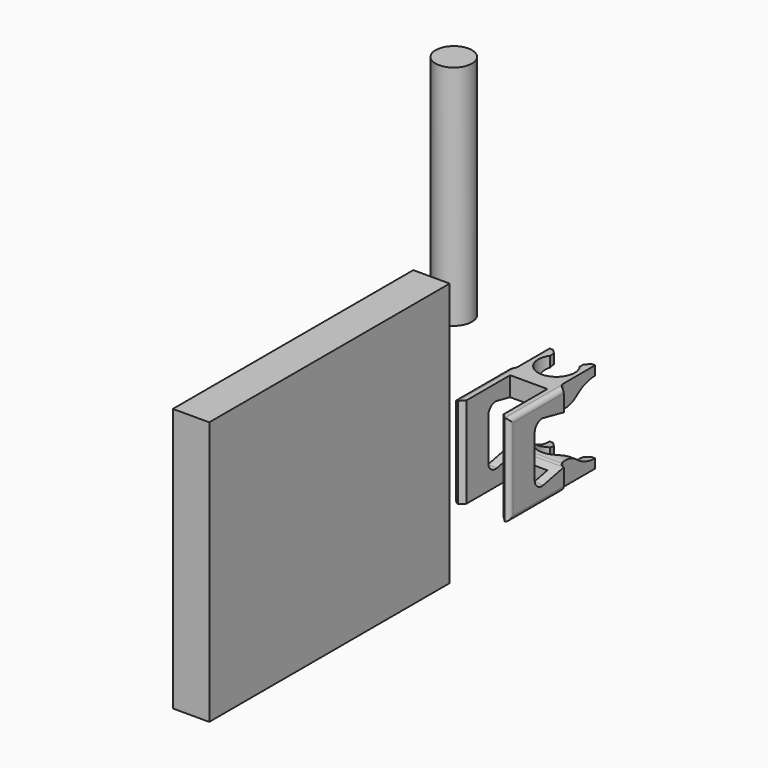
from build123d import *

# Parameters (mm, degrees)
F0_W        = 2
F0_H        = 20
F0_W_2      = 8.2
F1_DEPTH    = 15
F2_DEPTH    = 13
F3_W        = 10
F3_H        = 20
F4_DEPTH    = 10
F5_T1_DEPTH = 20
F7_DEPTH    = 20.001
F8_SIZE     = 1
F9_R        = 1
F10_SIZE    = 0.99999
F11_R       = 4
F12_DEPTH   = 50
F13_W       = 66.0741459578
F13_H       = 57.9895451665
F14_DEPTH   = 8
F16_DEPTH   = 25


# Not quite as in the source:
# - a fillet or chamfer that OpenCascade refuses, or shapes differently, is made with other operations: its cross-section is extruded or revolved along the edge and cut away or added
# - a fillet or chamfer is up to 0.001 mm smaller than in the source, because OpenCascade refuses the exact size
# - a feature names something its author has since deleted; it is built from what else it names


with BuildPart() as f1:
    # F0 (on Front) → F1 (new body)
    with BuildSketch(Plane.XZ):
        with Locations((1, 10)):
            Rectangle(F0_W, F0_H)
        with Locations((-9.2, 10)):
            Rectangle(F0_W, F0_H)
        with Locations((-4.1, 10)):
            Rectangle(F0_W_2, F0_H)
    extrude(amount=-F1_DEPTH)

    # F0 (on Front) → F2 (cut)
    with BuildSketch(Plane.XZ):
        with Locations((-4.1, 10)):
            Rectangle(F0_W_2, F0_H)
    extrude(amount=-F2_DEPTH, mode=Mode.SUBTRACT)

    # F3 (on face) → F4 (join)
    with BuildSketch(Plane(origin=(0, 15, 0), x_dir=(-1, 0, 0), z_dir=(0, 1, 0))):
        with Locations((4.1, 10)):
            Rectangle(F3_W, F3_H)
    extrude(amount=F4_DEPTH)

    # F5: fillet of radius 1.25 on 2 edges, made by hand

    # F5_s2 → F5_t1 (join)
    with BuildSketch(Plane.XY):
        with BuildLine():
            ThreePointArc((-10.2, 15), (-9.4145856533, 15.411811167), (-9.1, 16.2409673646))
            Line((-9.1, 16.2409673646), (-9.075, 16.2409673646))
            Line((-9.075, 16.2409673646), (-9.075, 15))
            Line((-9.075, 15), (-9.1, 14.975))
            ThreePointArc((-9.1, 14.975), (-9.65, 14.975), (-10.197, 14.9751806527))
            Line((-10.197, 14.9751806527), (-10.2, 15))
        make_face()
        with BuildLine():
            ThreePointArc((2, 15), (1.2145856533, 15.411811167), (0.9, 16.2409673646))
            Line((0.9, 16.2409673646), (0.875, 16.2409673646))
            Line((0.875, 16.2409673646), (0.875, 15))
            Line((0.875, 15), (0.9, 14.975))
            ThreePointArc((0.9, 14.975), (1.45, 14.975), (1.997, 14.9751806527))
            Line((1.997, 14.9751806527), (2, 15))
        make_face()
    extrude(amount=F5_T1_DEPTH)

    # F6 (on face) → F7 (cut, through all)
    with BuildSketch(Plane.XY.offset(20)):
        with BuildLine():
            Line((-7.35, 25), (-7.35, 22.9523284456))
            ThreePointArc((-7.35, 22.9523284456), (-4.1, 16.6204836823), (-0.85, 22.9523284456))
            Line((-0.85, 22.9523284456), (-0.85, 25))
            Line((-0.85, 25), (-7.35, 25))
        make_face()
    extrude(amount=-F7_DEPTH, mode=Mode.SUBTRACT)

    # F8
    f8_edges = [f1.edges().sort_by_distance(p)[0] for p in [
        (-0.85, 25, 10),
        (-7.35, 25, 10),
    ]]
    chamfer(f8_edges, length=F8_SIZE)

    # F9
    f9_edges = [f1.edges().sort_by_distance(p)[0] for p in [
        (-10.2, 7.5, 20),
        (-10.2, 7.5, 0),
        (-10.2, 0, 10),
        (2, 7.5, 20),
        (2, 7.5, 0),
        (2, 0, 10),
    ]]
    fillet(f9_edges, radius=F9_R)

    # F10 (size 1 in the source; OpenCascade refuses exactly that, so slightly less here)
    f10_edges = [f1.edges().sort_by_distance(p)[0] for p in [
        (0, 0, 10),
        (-8.2, 0, 10),
    ]]
    chamfer(f10_edges, length=F10_SIZE)

    # F15 (on face) → F16 (cut)
    with BuildSketch(Plane.YZ.offset(2)):
        with BuildLine():
            Line((15, 15.3167871196), (9.4117872498, 16.4925560795))
            ThreePointArc((9.4117872498, 16.4925560795), (7.7397568686, 16.0884003189), (7, 14.5354073216))
            Line((7, 14.5354073216), (7, 5.4645926784))
            ThreePointArc((7, 5.4645926784), (7.7397568686, 3.9115996811), (9.4117872498, 3.5074439205))
            Line((9.4117872498, 3.5074439205), (15, 4.6832128804))
            Line((15, 4.6832128804), (15, 15.3167871196))
        make_face()
        with BuildLine():
            Line((15.7314883663, 15.1628807896), (15, 15.3167871196))
            Line((15, 15.3167871196), (15, 4.6832128804))
            Line((15, 4.6832128804), (15.7314883663, 4.8371192104))
            ThreePointArc((15.7314883663, 4.8371192104), (17.9471476835, 4.8015048188), (19.9298193789, 3.8118445018))
            ThreePointArc((19.9298193789, 3.8118445018), (33, 10), (19.9298193789, 16.1881554982))
            ThreePointArc((19.9298193789, 16.1881554982), (17.9471476835, 15.1984951812), (15.7314883663, 15.1628807896))
        make_face()
    extrude(amount=-F16_DEPTH, mode=Mode.SUBTRACT)


with BuildPart() as f12:
    # F11 (on Top) → F12 (new body)
    with BuildSketch(Plane.XY):
        with Locations((-53.69772017, 54.3963909149)):
            Circle(F11_R)
    extrude(amount=F12_DEPTH)


with BuildPart() as f14:
    # F13 (on Right) → F14 (new body)
    with BuildSketch(Plane.YZ):
        with Locations((-56.8916359916, 28.9947725832)):
            Rectangle(F13_W, F13_H)
    extrude(amount=F14_DEPTH)


solid = Compound([f1.part, f12.part, f14.part])
